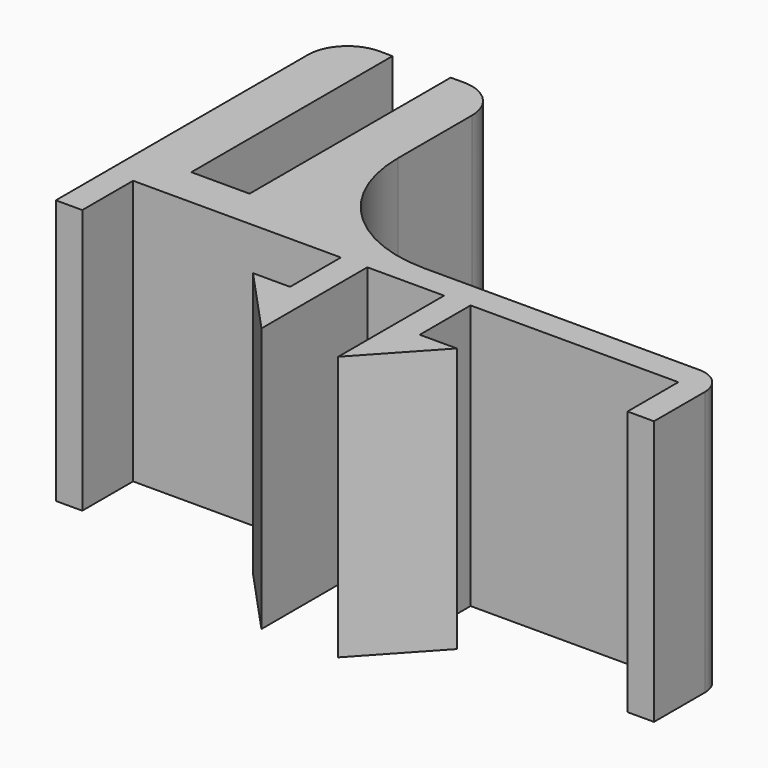
from build123d import *

# Parameters (mm, degrees)
F0_W     = 1
F0_H     = 2.4
F1_DEPTH = 10


# Not quite as in the source:
# - a feature names something its author has since deleted; it is built from what else it names


with BuildPart() as f1:
    # F0 (on Top) → F1 (new body)
    with BuildSketch(Plane.XY):
        with Locations((10.8, -6.7)):
            Rectangle(F0_W, F0_H)
        with Locations((-10.8, -6.7)):
            Rectangle(F0_W, F0_H)
        Polygon((-2.45, -8.5), (-2.45, -7.9), (-3.85, -7.9), (-1.45, -10.5), (-1.45, -8.5), align=None)
        with BuildLine():
            Line((10.3, -4.5), (10.3, -5.5))
            Line((10.3, -5.5), (11.3, -5.5))
            ThreePointArc((11.3, -5.5), (11.0071067812, -4.7928932188), (10.3, -4.5))
        make_face()
        Polygon((-1.45, -5.5), (-2.45, -5.5), (-2.45, -7.9), (-2.45, -8.5), (-1.45, -8.5), align=None)
        Polygon((2.45, -5.5), (1.45, -5.5), (1.45, -8.5), (2.45, -8.5), (2.45, -7.9), align=None)
        with BuildLine():
            Line((-11.3, -5.5), (-10.3, -5.5))
            Line((-10.3, -5.5), (-2.45, -5.5))
            Line((-2.45, -5.5), (-1.45, -5.5))
            Line((-1.45, -5.5), (1.45, -5.5))
            Line((1.45, -5.5), (2.45, -5.5))
            Line((2.45, -5.5), (10.3, -5.5))
            Line((10.3, -5.5), (10.3, -4.5))
            Line((10.3, -4.5), (-0.1, -4.5))
            ThreePointArc((-0.1, -4.5), (-3.6355339059, -3.0355339059), (-5.1, 0.5))
            Line((-5.1, 0.5), (-5.1, 4))
            ThreePointArc((-5.1, 4), (-5.5393398282, 5.0606601718), (-6.6, 5.5))
            Line((-6.6, 5.5), (-7.1, 5.5))
            Line((-7.1, 5.5), (-7.1, -4))
            Line((-7.1, -4), (-9.3, -4))
            Line((-9.3, -4), (-9.3, 5.5))
            Line((-9.3, 5.5), (-9.8, 5.5))
            ThreePointArc((-9.8, 5.5), (-10.8606601718, 5.0606601718), (-11.3, 4))
            Line((-11.3, 4), (-11.3, -5.5))
        make_face()
        Polygon((2.45, -8.5), (1.45, -8.5), (1.45, -10.5), (3.85, -7.9), (2.45, -7.9), align=None)
    extrude(amount=F1_DEPTH)


solid = f1.part
